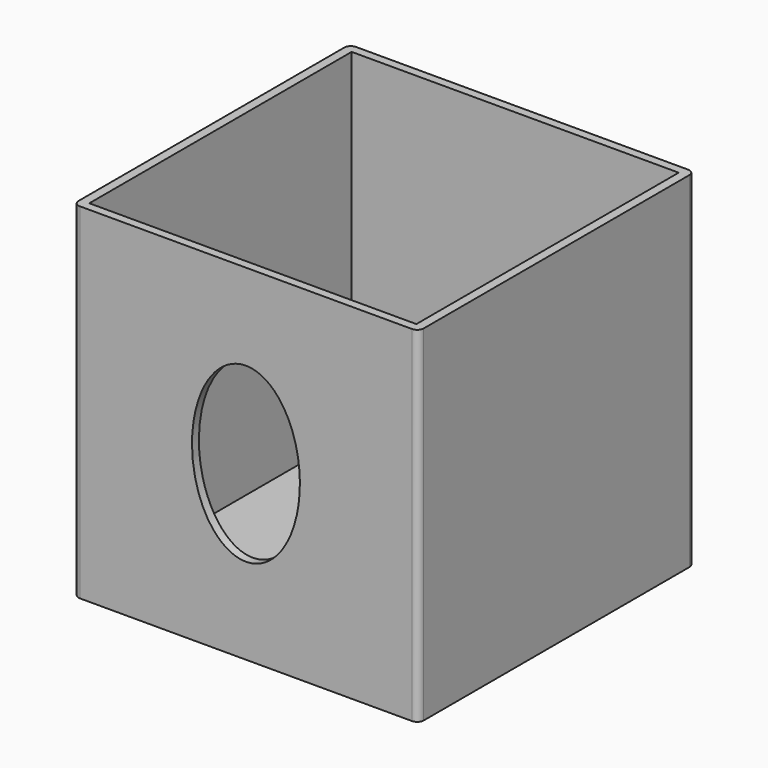
from build123d import *

# Parameters (mm, degrees)
F0_W     = 80
F0_H     = 80
F0_W_2   = 75.8
F0_H_2   = 76
F1_DEPTH = 80
F2_DEPTH = 2
F4_DEPTH = 25
F5_R     = 1.5


with BuildPart() as f1:
    # F0 (on Top) → F1 (new body)
    with BuildSketch(Plane.XY):
        Rectangle(F0_W, F0_H)
        Rectangle(F0_W_2, F0_H_2, mode=Mode.SUBTRACT)
    extrude(amount=F1_DEPTH)

    # F0 (on Top) → F2 (join)
    with BuildSketch(Plane.XY):
        Rectangle(F0_W_2, F0_H_2)
    extrude(amount=F2_DEPTH)

    # F3 (on face) → F4 (cut)
    with BuildSketch(Plane.XZ.offset(40)):
        with BuildLine():
            Line((0, 40), (0, 60))
            add(Edge.make_bspline(
                [(0, 60), (-12.5, 60), (-12.5, 40)],
                knots=[0, 0, 0, 1.5707963268, 1.5707963268, 1.5707963268], degree=2, weights=[1, 0.7071067812, 1]))
            Line((-12.5, 40), (0, 40))
        make_face()
        with BuildLine():
            add(Edge.make_bspline(
                [(12.5, 40), (12.5, 60), (0, 60)],
                knots=[4.7123889804, 4.7123889804, 4.7123889804, 6.2831853072, 6.2831853072, 6.2831853072], degree=2, weights=[1, 0.7071067812, 1]))
            Line((0, 60), (0, 40))
            Line((0, 40), (12.5, 40))
        make_face()
        with BuildLine():
            Line((12.5, 40), (0, 40))
            Line((0, 40), (0, 20))
            add(Edge.make_bspline(
                [(0, 20), (12.5, 20), (12.5, 40)],
                knots=[3.1415926536, 3.1415926536, 3.1415926536, 4.7123889804, 4.7123889804, 4.7123889804], degree=2, weights=[1, 0.7071067812, 1]))
        make_face()
        with BuildLine():
            Line((0, 20), (0, 40))
            Line((0, 40), (-12.5, 40))
            add(Edge.make_bspline(
                [(-12.5, 40), (-12.5, 20), (0, 20)],
                knots=[1.5707963268, 1.5707963268, 1.5707963268, 3.1415926536, 3.1415926536, 3.1415926536], degree=2, weights=[1, 0.7071067812, 1]))
        make_face()
    extrude(amount=-F4_DEPTH, mode=Mode.SUBTRACT)

    # F5
    f5_edges = [f1.edges().sort_by_distance(p)[0] for p in [
        (-40, -40, 40),
        (40, 40, 40),
        (-40, 40, 40),
        (40, -40, 40),
    ]]
    fillet(f5_edges, radius=F5_R)


solid = f1.part
